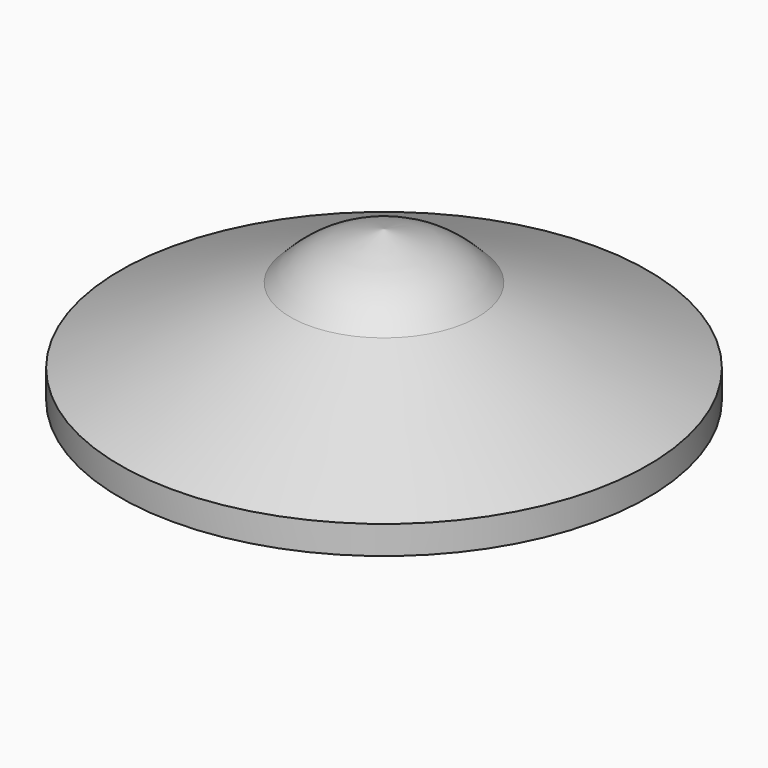
from build123d import *

# Parameters (mm, degrees)
F2_R            = 16.51
F3_DEPTH        = 4.7625
F4_R            = 12.7
F5_DEPTH        = 12.7
F6_R            = 3.81
F7_DEPTH        = 2.54
F7_COPIES_COUNT = 12


# Not quite as in the source:
# - a pattern or mirror of a feature is missing from the dataset's text; its kind, count and spacing are read off the source's solid


with BuildPart() as f1:
    # F0 (on Right) → F1 (revolve)
    with BuildSketch(Plane.YZ):
        with BuildLine():
            Line((0, 25.4), (0, 0))
            Line((0, 0), (44.4412930132, 0))
            Line((44.4412930132, 0), (44.4412930132, 4.7663409987))
            Line((44.4412930132, 4.7663409987), (15.7640874386, 17.416998744))
            add(Edge.make_bspline(
                [(0, 25.4), (3.7261787695, 24.441300081), (10.4835897095, 22.7027014465), (14.128884846, 19.0538131517), (15.7640874386, 17.416998744)],
                knots=[0, 0, 0, 0, 0.5514210698, 1, 1, 1, 1], degree=3))
        make_face()
    revolve(axis=Axis((0, 0, 12.7), (0, 0, -1)))

    # F2 (on face) → F3 (cut)
    with BuildSketch(Plane(origin=(0, 0, 0), x_dir=(1, 0, 0), z_dir=(0, 0, -1))):
        Circle(F2_R)
    extrude(amount=-F3_DEPTH, mode=Mode.SUBTRACT)

    # F4 (on face) → F5 (cut)
    with BuildSketch(Plane(origin=(0, 0, 4.7625), x_dir=(1, 0, 0), z_dir=(0, 0, -1))):
        Circle(F4_R)
    extrude(amount=-F5_DEPTH, mode=Mode.SUBTRACT)

    # F6 (on face) → F7 (cut)
    with BuildSketch(Plane(origin=(0, 0, 0), x_dir=(1, 0, 0), z_dir=(0, 0, -1))):
        with Locations((0, 35.0116197045)):
            Circle(F6_R)
    f7 = extrude(amount=-F7_DEPTH, mode=Mode.SUBTRACT)

    # F7_copies: F7 ×12 about axis
    f7_copies_axis = Axis((0, 0, 0), (0, 0, 1))
    for i in range(1, F7_COPIES_COUNT):
        add(f7.rotate(f7_copies_axis, i * 360 / F7_COPIES_COUNT), mode=Mode.SUBTRACT)


solid = f1.part
